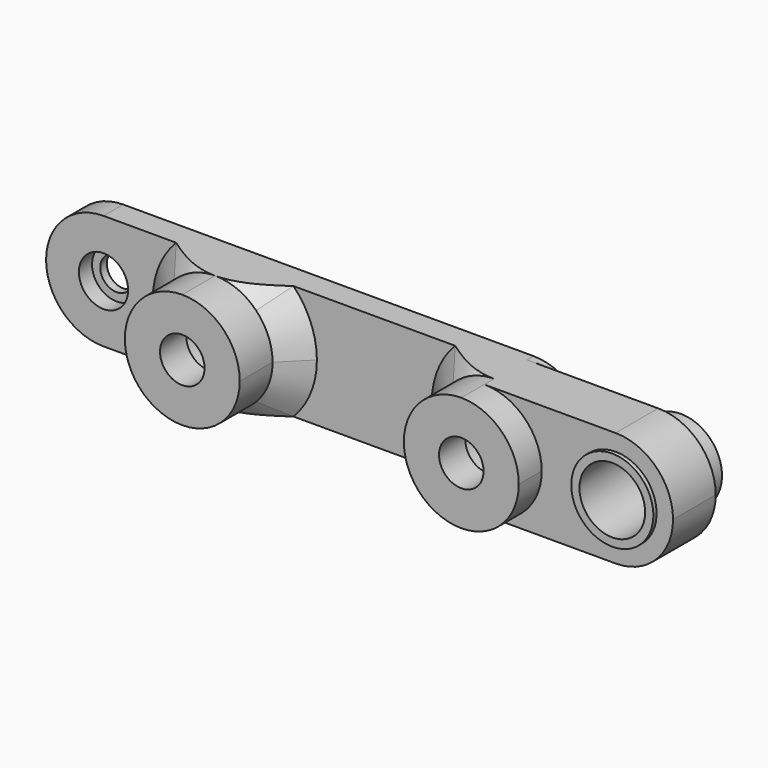
from build123d import *

# Parameters (mm, degrees)
F1_DEPTH      = 11.1125
F2_R          = 3.175
F2_R_2        = 1.5875
F2_R_3        = 2.15265
F3_DEPTH      = 8.73125
F4_R          = 2.38125
F5_DEPTH      = 1.5875
F6_R          = 3.96875
F6_R_2        = 3.175
F7_DEPTH      = 2.746375
F7_DEPTH_BACK = 5.55625
F8_R          = 5.55624
F10_R         = 3.96875
F11_DEPTH     = 5.55625
F12_C1_SIZE   = 2.38125
F12_C2_SIZE   = 2.38125
F12_C3_SIZE   = 2.38125


# Not quite as in the source:
# - a fillet or chamfer is up to 0.001 mm smaller than in the source, because OpenCascade refuses the exact size


with BuildPart() as f1:
    # F0 (on Top) → F1 (new body)
    with BuildSketch(Plane.XY):
        Polygon((-12.7, 0), (0, 0), (0, -6.35), (11.1125, -6.35), (11.1125, 0), (26.9875, 0), (26.9875, -6.35), (38.1, -6.35), (38.1, -3.571875), (50.8, -3.571875), (50.8, 1.5875), (38.1, 1.5875), (38.1, 2.38125), (-12.7, 2.38125), align=None)
    extrude(amount=F1_DEPTH)

    # F2 (on face) → F3 (cut, through all)
    with BuildSketch(Plane(origin=(0, 2.38125, 0), x_dir=(-1, 0, 0), z_dir=(0, 1, 0))):
        with Locations((-45.24375, 5.55625)):
            Circle(F2_R)
        with Locations((7.14375, 5.55625)):
            Circle(F2_R_2)
        with Locations((-5.55625, 5.55625)):
            Circle(F2_R_3)
        with Locations((-32.54375, 5.55625)):
            Circle(F2_R_3)
    extrude(amount=-F3_DEPTH, mode=Mode.SUBTRACT)

    # F4 (on face) → F5 (cut)
    with BuildSketch(Plane.XZ):
        with Locations((-7.14375, 5.55625)):
            Circle(F4_R)
    extrude(amount=-F5_DEPTH, mode=Mode.SUBTRACT)

    # F6 (on face) → F7 (join, two sides)
    with BuildSketch(Plane(origin=(0, 1.5875, 0), x_dir=(-1, 0, 0), z_dir=(0, 1, 0))) as f7_sk:
        with Locations((-45.24375, 5.55625)):
            Circle(F6_R)
        with Locations((-45.24375, 5.55625)):
            Circle(F6_R_2, mode=Mode.SUBTRACT)
    extrude(amount=F7_DEPTH)
    extrude(f7_sk.sketch, amount=-F7_DEPTH_BACK)

    # F8 (radius 5.55625 in the source; OpenCascade refuses exactly that, so slightly less here)
    f8_edges = [f1.edges().sort_by_distance(p)[0] for p in [
        (0, -3.175, 0),
        (0, -3.175, 11.1125),
        (38.1, -4.960938, 0),
        (38.1, -4.960938, 11.1125),
        (38.1, 1.984375, 0),
        (38.1, 1.984375, 11.1125),
        (11.1125, -3.175, 11.1125),
        (11.1125, -3.175, 0),
        (26.9875, -3.175, 11.1125),
        (26.9875, -3.175, 0),
        (50.8, -0.992188, 11.1125),
        (50.8, -0.992188, 0),
        (-12.7, 1.190625, 11.1125),
        (-12.7, 1.190625, 0),
    ]]
    fillet(f8_edges, radius=F8_R)

    # F10 (on face) → F11 (cut, through all)
    with BuildSketch(Plane(origin=(0, 2.38125, 0), x_dir=(-1, 0, 0), z_dir=(0, 1, 0))):
        with Locations((-32.54375, 5.55625)):
            Circle(F10_R)
        with Locations((-5.55625, 5.55625)):
            Circle(F10_R)
    extrude(amount=-F11_DEPTH, mode=Mode.SUBTRACT)

    # F12: chamfer of 2.38125 on 5 edges, made by hand

    # F12_c1
    f12_c1_edges = [f1.edges().sort_by_distance(p)[0] for p in [
        (1.6273850181, 0, 9.4851149819),
        (0, 0, 5.55625),
        (1.6273850181, 0, 1.6273850181),
    ]]
    chamfer(f12_c1_edges, length=F12_C1_SIZE)

    # F12_c2
    f12_c2_edges = [f1.edges().sort_by_distance(p)[0] for p in [
        (28.6148850181, 0, 9.4851149819),
        (26.9875, 0, 5.55625),
        (28.6148850181, 0, 1.6273850181),
    ]]
    chamfer(f12_c2_edges, length=F12_C2_SIZE)

    # F12_c3
    f12_c3_edges = [f1.edges().sort_by_distance(p)[0] for p in [
        (11.1125, 0, 5.55625),
        (9.4851149819, 0, 9.4851149819),
        (9.4851149819, 0, 1.6273850181),
    ]]
    chamfer(f12_c3_edges, length=F12_C3_SIZE)


solid = f1.part
